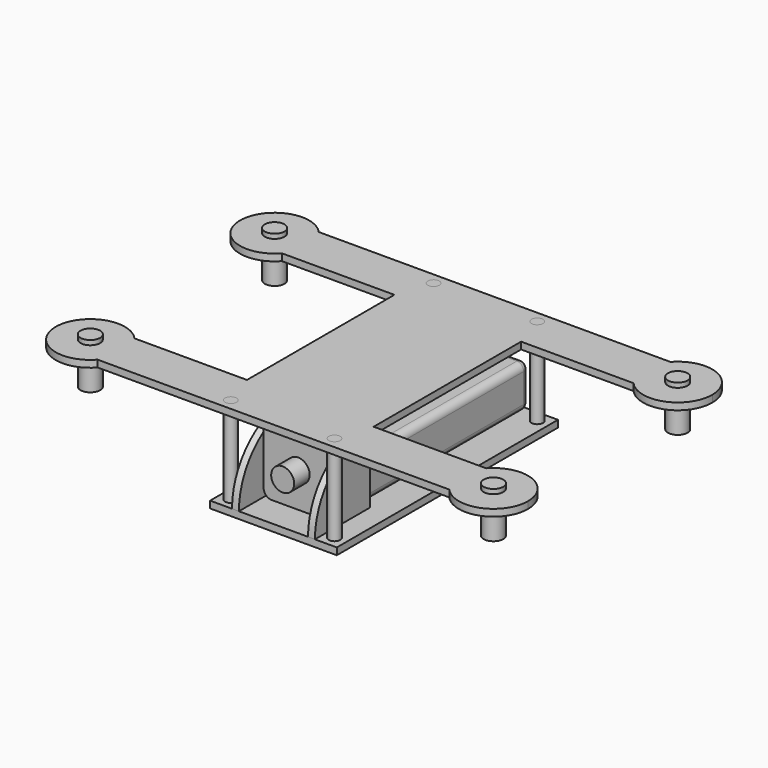
from build123d import *

# Parameters (mm, degrees)
F2_R          = 2.5
F2_R_2        = 4.25
F3_DEPTH      = 3
F0_R          = 2.5
F4_DEPTH      = 3
F5_DEPTH      = 38
F5_DEPTH_BACK = 3
F6_DEPTH      = 5
F6_DEPTH_BACK = 15
F8_DEPTH      = 18
F9_DEPTH      = 15
F12_START     = 15
F11_R         = 5
F12_DEPTH     = 1.6
F13_START     = 15
F13_DEPTH     = 10
F14_R         = 3.5
F15_DEPTH     = 18.6
F16_R         = 3


with BuildPart() as f3:
    # F2 (on offset) → F3 (new body)
    with BuildSketch(Plane.XY.offset(35)):
        Polygon((-27.5, -60), (27.5, -60), (27.5, -40), (27.5, 40), (27.5, 60), (-27.5, 60), (-27.5, 55), (-27.5, 40), (-27.5, -40), align=None)
        with Locations((-22.5, -55)):
            Circle(F2_R, mode=Mode.SUBTRACT)
        with Locations((22.5, -55)):
            Circle(F2_R, mode=Mode.SUBTRACT)
        with Locations((-22.5, 55)):
            Circle(F2_R, mode=Mode.SUBTRACT)
        with Locations((22.5, 55)):
            Circle(F2_R, mode=Mode.SUBTRACT)
        with BuildLine():
            Line((27.5, -40), (27.5, -60))
            Line((27.5, -60), (76.3196601125, -60))
            ThreePointArc((76.3196601125, -60), (72.5, -50), (76.3196601125, -40))
            Line((76.3196601125, -40), (27.5, -40))
        make_face()
        with BuildLine():
            Line((-76.3196601125, -60), (-27.5, -60))
            Line((-27.5, -60), (-27.5, -40))
            Line((-27.5, -40), (-76.3196601125, -40))
            ThreePointArc((-76.3196601125, -40), (-73.4874146156, -44.6476686534), (-72.5, -50))
            ThreePointArc((-72.5, -50), (-73.4874146156, -55.3523313466), (-76.3196601125, -60))
        make_face()
        with BuildLine():
            ThreePointArc((76.3196601125, -40), (72.5, -50), (76.3196601125, -60))
            ThreePointArc((76.3196601125, -60), (92.8523313466, -64.0125853844), (102.5, -50))
            ThreePointArc((102.5, -50), (92.8523313466, -35.9874146156), (76.3196601125, -40))
        make_face()
        with Locations((87.5, -50)):
            Circle(F2_R_2, mode=Mode.SUBTRACT)
        with BuildLine():
            ThreePointArc((-76.3196601125, -40), (-102.5, -50), (-76.3196601125, -60))
            ThreePointArc((-76.3196601125, -60), (-73.4874146156, -55.3523313466), (-72.5, -50))
            ThreePointArc((-72.5, -50), (-73.4874146156, -44.6476686534), (-76.3196601125, -40))
        make_face()
        with Locations((-87.5, -50)):
            Circle(F2_R_2, mode=Mode.SUBTRACT)
        with BuildLine():
            Line((27.5, 60), (27.5, 40))
            Line((27.5, 40), (76.3196601125, 40))
            ThreePointArc((76.3196601125, 40), (72.5, 50), (76.3196601125, 60))
            Line((76.3196601125, 60), (27.5, 60))
        make_face()
        with BuildLine():
            Line((-76.3196601125, 40), (-27.5, 40))
            Line((-27.5, 40), (-27.5, 55))
            Line((-27.5, 55), (-27.5, 60))
            Line((-27.5, 60), (-76.3196601125, 60))
            ThreePointArc((-76.3196601125, 60), (-73.4874146156, 55.3523313466), (-72.5, 50))
            ThreePointArc((-72.5, 50), (-73.4874146156, 44.6476686534), (-76.3196601125, 40))
        make_face()
        with BuildLine():
            ThreePointArc((76.3196601125, 60), (72.5, 50), (76.3196601125, 40))
            ThreePointArc((76.3196601125, 40), (92.8523313466, 35.9874146156), (102.5, 50))
            ThreePointArc((102.5, 50), (92.8523313466, 64.0125853844), (76.3196601125, 60))
        make_face()
        with Locations((87.5, 50)):
            Circle(F2_R_2, mode=Mode.SUBTRACT)
        with BuildLine():
            ThreePointArc((-76.3196601125, 60), (-102.5, 50), (-76.3196601125, 40))
            ThreePointArc((-76.3196601125, 40), (-73.4874146156, 44.6476686534), (-72.5, 50))
            ThreePointArc((-72.5, 50), (-73.4874146156, 55.3523313466), (-76.3196601125, 60))
        make_face()
        with Locations((-87.5, 50)):
            Circle(F2_R_2, mode=Mode.SUBTRACT)
    extrude(amount=F3_DEPTH)


with BuildPart() as f4:
    # F0 (on Top) → F4 (new body)
    with BuildSketch(Plane.XY):
        Polygon((-27.5, -60), (27.5, -60), (27.5, 60), (15, 60), (15, -30), (-15, -30), (-15, 60), (-27.5, 60), (-27.5, 55), align=None)
        with Locations((-22.5, -55)):
            Circle(F0_R, mode=Mode.SUBTRACT)
        with Locations((22.5, -55)):
            Circle(F0_R, mode=Mode.SUBTRACT)
        with Locations((-22.5, 55)):
            Circle(F0_R, mode=Mode.SUBTRACT)
        with Locations((22.5, 55)):
            Circle(F0_R, mode=Mode.SUBTRACT)
        Polygon((15, -30), (15, 60), (0, 60), (-15, 60), (-15, -30), align=None)
    extrude(amount=-F4_DEPTH)

    # F7 (on Right) → F8 (join, symmetric)
    with BuildSketch(Plane.YZ):
        with BuildLine():
            Line((-60, 0), (-30, 0))
            Line((-30, 0), (-30, 30))
            ThreePointArc((-30, 30), (-51.2132034356, 21.2132034356), (-60, 0))
        make_face()
    extrude(amount=F8_DEPTH, both=True)

    # F7 (on Right) → F9 (cut, symmetric)
    with BuildSketch(Plane.YZ):
        with BuildLine():
            Line((-60, 0), (-30, 0))
            Line((-30, 0), (-30, 30))
            ThreePointArc((-30, 30), (-51.2132034356, 21.2132034356), (-60, 0))
        make_face()
    extrude(amount=F9_DEPTH, both=True, mode=Mode.SUBTRACT)


with BuildPart() as f5:
    # F0 (on Top) → F5 (new body, two sides)
    with BuildSketch(Plane.XY) as f5_sk:
        with Locations((-22.5, 55)):
            Circle(F0_R)
    extrude(amount=F5_DEPTH)
    extrude(f5_sk.sketch, amount=-F5_DEPTH_BACK)


with BuildPart() as f5b:
    # F0 (on Top) → F5, piece 2 (new body, two sides)
    with BuildSketch(Plane.XY) as f5_2_sk:
        with Locations((22.5, 55)):
            Circle(F0_R)
    extrude(amount=F5_DEPTH)
    extrude(f5_2_sk.sketch, amount=-F5_DEPTH_BACK)


with BuildPart() as f5c:
    # F0 (on Top) → F5, piece 3 (new body, two sides)
    with BuildSketch(Plane.XY) as f5_3_sk:
        with Locations((22.5, -55)):
            Circle(F0_R)
    extrude(amount=F5_DEPTH)
    extrude(f5_3_sk.sketch, amount=-F5_DEPTH_BACK)


with BuildPart() as f5d:
    # F0 (on Top) → F5, piece 4 (new body, two sides)
    with BuildSketch(Plane.XY) as f5_4_sk:
        with Locations((-22.5, -55)):
            Circle(F0_R)
    extrude(amount=F5_DEPTH)
    extrude(f5_4_sk.sketch, amount=-F5_DEPTH_BACK)


with BuildPart() as f6:
    # F2 (on offset) → F6 (new body, two sides)
    with BuildSketch(Plane.XY.offset(35)) as f6_sk:
        with Locations((-87.5, -50)):
            Circle(F2_R_2)
    extrude(amount=F6_DEPTH)
    extrude(f6_sk.sketch, amount=-F6_DEPTH_BACK)


with BuildPart() as f6b:
    # F2 (on offset) → F6, piece 2 (new body, two sides)
    with BuildSketch(Plane.XY.offset(35)) as f6_2_sk:
        with Locations((87.5, -50)):
            Circle(F2_R_2)
    extrude(amount=F6_DEPTH)
    extrude(f6_2_sk.sketch, amount=-F6_DEPTH_BACK)


with BuildPart() as f6c:
    # F2 (on offset) → F6, piece 3 (new body, two sides)
    with BuildSketch(Plane.XY.offset(35)) as f6_3_sk:
        with Locations((-87.5, 50)):
            Circle(F2_R_2)
    extrude(amount=F6_DEPTH)
    extrude(f6_3_sk.sketch, amount=-F6_DEPTH_BACK)


with BuildPart() as f6d:
    # F2 (on offset) → F6, piece 4 (new body, two sides)
    with BuildSketch(Plane.XY.offset(35)) as f6_4_sk:
        with Locations((87.5, 50)):
            Circle(F2_R_2)
    extrude(amount=F6_DEPTH)
    extrude(f6_4_sk.sketch, amount=-F6_DEPTH_BACK)


with BuildPart() as f12:
    # F11 (on line) → F12 (new body)
    with BuildSketch(Plane.XZ.offset(30).offset(F12_START)):
        Polygon((-15, 0), (0, 0), (15, 0), (15, 30), (-15, 30), align=None)
        with Locations((0, 15)):
            Circle(F11_R, mode=Mode.SUBTRACT)
        with Locations((0, 15)):
            Circle(F11_R)
    extrude(amount=F12_DEPTH)

    # F11 (on line) → F13 (join)
    with BuildSketch(Plane.XZ.offset(30).offset(F13_START)):
        with Locations((0, 15)):
            Circle(F11_R)
    extrude(amount=F13_DEPTH)

    # F14
    f14_edges = [f12.edges().sort_by_distance(p)[0] for p in [
        (-15, -45.8, 0),
        (-15, -45.8, 30),
        (15, -45.8, 30),
        (15, -45.8, 0),
    ]]
    fillet(f14_edges, radius=F14_R)


with BuildPart() as f15:
    # F0 (on Top) → F15 (new body)
    with BuildSketch(Plane.XY):
        Polygon((15, -30), (15, 60), (0, 60), (-15, 60), (-15, -30), align=None)
    extrude(amount=F15_DEPTH)

    # F16
    f16_edges = [f15.edges().sort_by_distance(p)[0] for p in [
        (15, 15, 18.6),
        (0, -30, 18.6),
        (-15, 15, 18.6),
        (0, 60, 18.6),
        (-15, 60, 9.3),
        (15, 60, 9.3),
        (15, -30, 9.3),
        (15, 15, 0),
        (0, 60, 0),
        (0, -30, 0),
        (-15, -30, 9.3),
        (-15, 15, 0),
    ]]
    fillet(f16_edges, radius=F16_R)


solid = Compound([f3.part, f4.part, f5.part, f5b.part, f5c.part, f5d.part, f6.part, f6b.part, f6c.part, f6d.part, f12.part, f15.part])
